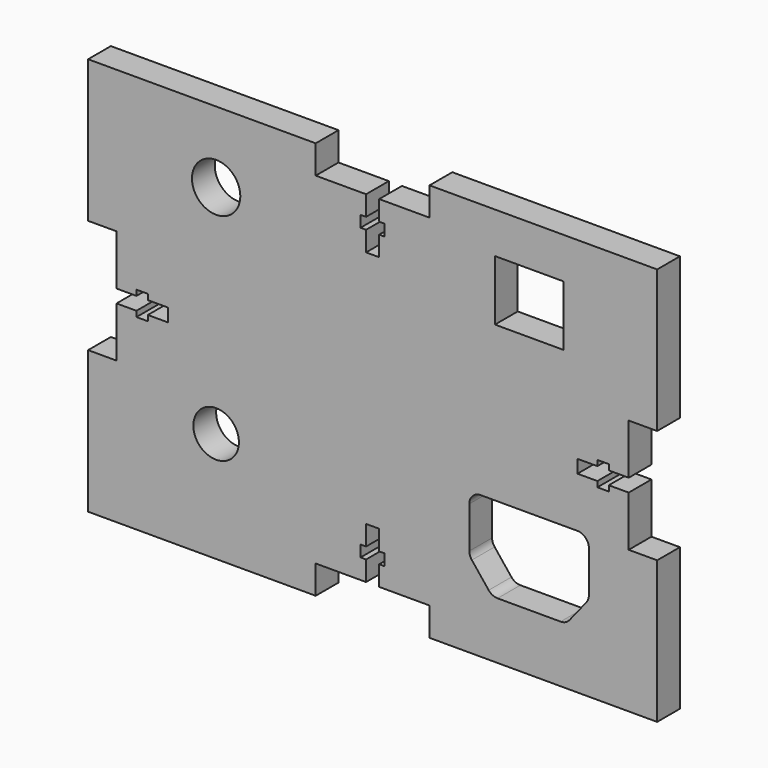
from build123d import *

# Parameters (mm, degrees)
F0_R     = 5.08
F0_R_2   = 5.3975
F1_DEPTH = 6.35


# Not quite as in the source:
# - a feature names something its author has since deleted; it is built from what else it names


with BuildPart() as f1:
    # F0 (on Front) → F1 (new body)
    with BuildSketch(Plane.XZ):
        with BuildLine():
            Line((34.9250002354, -44.45), (57.1500004709, -44.45))
            Line((57.1500004709, -44.45), (63.5, -44.45))
            Line((63.5, -44.45), (63.5, -12.7))
            Line((63.5, -12.7), (57.1500004709, -12.7))
            Line((57.1500004709, -12.7), (57.1500004709, -1.4605))
            Line((57.1500004709, -1.4605), (52.7050002354, -1.4605))
            Line((52.7050002354, -1.4605), (52.7050002354, -2.69367))
            Line((52.7050002354, -2.69367), (50.1650002354, -2.69367))
            Line((50.1650002354, -2.69367), (50.1650002354, -1.4605))
            Line((50.1650002354, -1.4605), (45.72, -1.4605))
            Line((45.72, -1.4605), (45.72, 1.4605))
            Line((45.72, 1.4605), (50.1650002354, 1.4605))
            Line((50.1650002354, 1.4605), (50.1650002354, 2.69367))
            Line((50.1650002354, 2.69367), (52.7050002354, 2.69367))
            Line((52.7050002354, 2.69367), (52.7050002354, 1.4605))
            Line((52.7050002354, 1.4605), (57.1500004709, 1.4605))
            Line((57.1500004709, 1.4605), (57.1500004709, 12.7))
            Line((57.1500004709, 12.7), (63.5, 12.7))
            Line((63.5, 12.7), (63.5, 44.45))
            Line((63.5, 44.45), (57.1500004709, 44.45))
            Line((57.1500004709, 44.45), (34.9250002354, 44.45))
            Line((34.9250002354, 44.45), (34.9250002354, 35.306))
            Line((34.9250002354, 35.306), (42.5450002354, 35.306))
            Line((42.5450002354, 35.306), (42.5450002354, 21.844))
            Line((42.5450002354, 21.844), (34.9250002354, 21.844))
            Line((34.9250002354, 21.844), (34.9250002354, -12.7))
            Line((34.9250002354, -12.7), (45.7200002354, -12.7))
            ThreePointArc((45.7200002354, -12.7), (47.5160514597, -13.4439487758), (48.2600002354, -15.24))
            Line((48.2600002354, -15.24), (48.2600002354, -24.5090161092))
            ThreePointArc((48.2600002354, -24.5090161092), (48.1168161661, -25.3497737405), (47.7034070114, -26.09574153))
            Line((47.7034070114, -26.09574153), (43.9426198988, -30.7967254208))
            ThreePointArc((43.9426198988, -30.7967254208), (43.0595124983, -31.4993102202), (41.9592131228, -31.75))
            Line((41.9592131228, -31.75), (34.9250002354, -31.75))
            Line((34.9250002354, -31.75), (34.9250002354, -44.45))
        make_face()
        with BuildLine():
            Line((12.7, -44.45), (34.9250002354, -44.45))
            Line((34.9250002354, -44.45), (34.9250002354, -31.75))
            Line((34.9250002354, -31.75), (27.8907873481, -31.75))
            ThreePointArc((27.8907873481, -31.75), (26.7904879726, -31.4993102202), (25.9073805721, -30.7967254208))
            Line((25.9073805721, -30.7967254208), (22.1465934595, -26.09574153))
            ThreePointArc((22.1465934595, -26.09574153), (21.7331843048, -25.3497737405), (21.5900002354, -24.5090161092))
            Line((21.5900002354, -24.5090161092), (21.5900002354, -15.24))
            ThreePointArc((21.5900002354, -15.24), (22.3339490112, -13.4439487758), (24.1300002354, -12.7))
            Line((24.1300002354, -12.7), (34.9250002354, -12.7))
            Line((34.9250002354, -12.7), (34.9250002354, 21.844))
            Line((34.9250002354, 21.844), (27.3050002354, 21.844))
            Line((27.3050002354, 21.844), (27.3050002354, 35.306))
            Line((27.3050002354, 35.306), (34.9250002354, 35.306))
            Line((34.9250002354, 35.306), (34.9250002354, 44.45))
            Line((34.9250002354, 44.45), (12.7, 44.45))
            Line((12.7, 44.45), (12.7, 38.1000004709))
            Line((12.7, 38.1000004709), (1.4605, 38.1000004709))
            Line((1.4605, 38.1000004709), (1.4605, 33.6550002354))
            Line((1.4605, 33.6550002354), (2.69367, 33.6550002354))
            Line((2.69367, 33.6550002354), (2.69367, 31.1150002354))
            Line((2.69367, 31.1150002354), (1.4605, 31.1150002354))
            Line((1.4605, 31.1150002354), (1.4605, 26.67))
            Line((1.4605, 26.67), (-1.4605, 26.67))
            Line((-1.4605, 26.67), (-1.4605, 31.1150002354))
            Line((-1.4605, 31.1150002354), (-2.69367, 31.1150002354))
            Line((-2.69367, 31.1150002354), (-2.69367, 33.6550002354))
            Line((-2.69367, 33.6550002354), (-1.4605, 33.6550002354))
            Line((-1.4605, 33.6550002354), (-1.4605, 38.1000004709))
            Line((-1.4605, 38.1000004709), (-12.7, 38.1000004709))
            Line((-12.7, 38.1000004709), (-12.7, 44.45))
            Line((-12.7, 44.45), (-57.1500004709, 44.45))
            Line((-57.1500004709, 44.45), (-63.5, 44.45))
            Line((-63.5, 44.45), (-63.5, 12.7))
            Line((-63.5, 12.7), (-57.1500004709, 12.7))
            Line((-57.1500004709, 12.7), (-57.1500004709, 1.4605))
            Line((-57.1500004709, 1.4605), (-52.7050002354, 1.4605))
            Line((-52.7050002354, 1.4605), (-52.7050002354, 2.69367))
            Line((-52.7050002354, 2.69367), (-50.1650002354, 2.69367))
            Line((-50.1650002354, 2.69367), (-50.1650002354, 1.4605))
            Line((-50.1650002354, 1.4605), (-45.72, 1.4605))
            Line((-45.72, 1.4605), (-45.72, -1.4605))
            Line((-45.72, -1.4605), (-50.1650002354, -1.4605))
            Line((-50.1650002354, -1.4605), (-50.1650002354, -2.69367))
            Line((-50.1650002354, -2.69367), (-52.7050002354, -2.69367))
            Line((-52.7050002354, -2.69367), (-52.7050002354, -1.4605))
            Line((-52.7050002354, -1.4605), (-57.1500004709, -1.4605))
            Line((-57.1500004709, -1.4605), (-57.1500004709, -2.69367))
            Line((-57.1500004709, -2.69367), (-57.1500004709, -12.7))
            Line((-57.1500004709, -12.7), (-63.5, -12.7))
            Line((-63.5, -12.7), (-63.5, -44.45))
            Line((-63.5, -44.45), (-57.1500004709, -44.45))
            Line((-57.1500004709, -44.45), (-12.7, -44.45))
            Line((-12.7, -44.45), (-12.7, -38.1000004709))
            Line((-12.7, -38.1000004709), (-1.4605, -38.1000004709))
            Line((-1.4605, -38.1000004709), (-1.4605, -33.6550002354))
            Line((-1.4605, -33.6550002354), (-2.69367, -33.6550002354))
            Line((-2.69367, -33.6550002354), (-2.69367, -31.1150002354))
            Line((-2.69367, -31.1150002354), (-1.4605, -31.1150002354))
            Line((-1.4605, -31.1150002354), (-1.4605, -26.67))
            Line((-1.4605, -26.67), (1.4605, -26.67))
            Line((1.4605, -26.67), (1.4605, -31.1150002354))
            Line((1.4605, -31.1150002354), (2.69367, -31.1150002354))
            Line((2.69367, -31.1150002354), (2.69367, -33.6550002354))
            Line((2.69367, -33.6550002354), (1.4605, -33.6550002354))
            Line((1.4605, -33.6550002354), (1.4605, -38.1000004709))
            Line((1.4605, -38.1000004709), (12.7, -38.1000004709))
            Line((12.7, -38.1000004709), (12.7, -44.45))
        make_face()
        with Locations((-34.9250002354, -19.8745080546)):
            Circle(F0_R, mode=Mode.SUBTRACT)
        with Locations((-34.9250002354, 28.575)):
            Circle(F0_R_2, mode=Mode.SUBTRACT)
    extrude(amount=F1_DEPTH)


solid = f1.part
